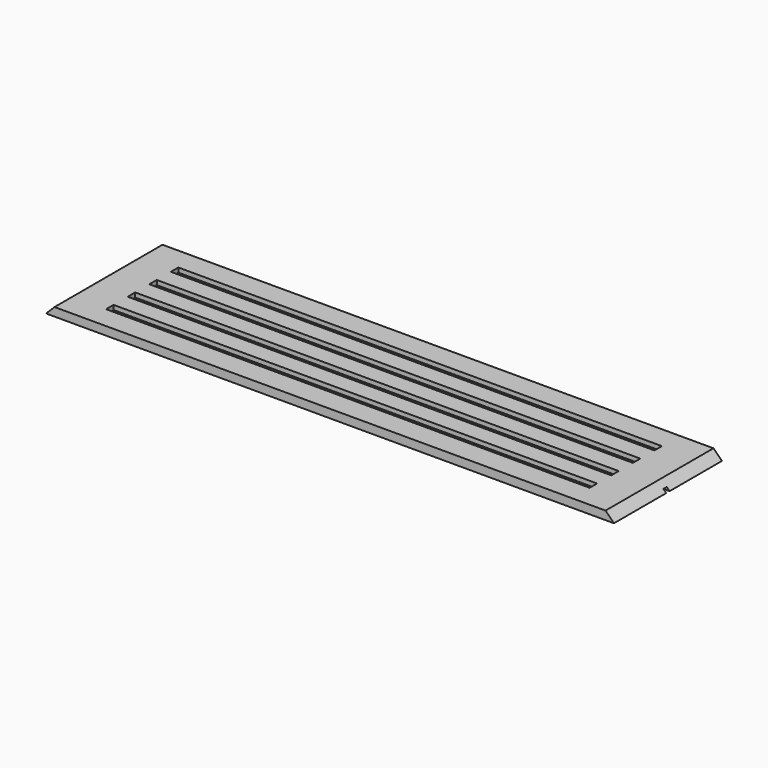
from build123d import *

# Parameters (mm, degrees)
F0_W     = 1282.7
F0_H     = 304.8
F1_DEPTH = 19.05
F2_SIZE  = 19.04999
F3_W     = 1092.2
F3_H     = 21.082
F4_DEPTH = 10.16
F6_DEPTH = 6.35


# Not quite as in the source:
# - a fillet or chamfer is up to 0.001 mm smaller than in the source, because OpenCascade refuses the exact size


with BuildPart() as f1:
    # F0 (on Top) → F1 (new body)
    with BuildSketch(Plane.XY):
        with Locations((362.7905342946, -3.9232242852)):
            Rectangle(F0_W, F0_H)
    extrude(amount=F1_DEPTH)

    # F2 (size 19.05 in the source; OpenCascade refuses exactly that, so slightly less here)
    f2_edges = [f1.edges().sort_by_distance(p)[0] for p in [
        (1004.140534, -3.923224, 19.05),
        (-278.559466, -3.923224, 19.05),
    ]]
    chamfer(f2_edges, length=F2_SIZE)

    # F3 (on face) → F4 (cut)
    with BuildSketch(Plane.XY.offset(19.05)):
        with Locations((362.7905342946, 87.5167757148)):
            Rectangle(F3_W, F3_H)
        with Locations((362.7905342946, 26.5567757148)):
            Rectangle(F3_W, F3_H)
        with Locations((362.7905342946, -34.4032242852)):
            Rectangle(F3_W, F3_H)
        with Locations((362.7905342946, -95.3632242852)):
            Rectangle(F3_W, F3_H)
    extrude(amount=-F4_DEPTH, mode=Mode.SUBTRACT)

    # F5 (on face) → F6 (cut)
    with BuildSketch(Plane(origin=(0, 0, 0), x_dir=(1, 0, 0), z_dir=(0, 0, -1))):
        Polygon((899.3655342946, 105.9042242852), (899.3655342946, -98.0577757148), (908.8905342946, -98.0577757148), (908.8905342946, -0.8392757148), (1004.1405342946, -0.8392757148), (1004.1405342946, 8.6857242852), (908.8905342946, 8.6857242852), (908.8905342946, 105.9042242852), align=None)
        Polygon((-278.5594657054, 8.6857242852), (-278.5594657054, -0.8392757148), (-183.3094657054, -0.8392757148), (-183.3094657054, -98.0577757148), (-173.7844657054, -98.0577757148), (-173.7844657054, 105.9042242852), (-183.3094657054, 105.9042242852), (-183.3094657054, 8.6857242852), align=None)
    extrude(amount=-F6_DEPTH, mode=Mode.SUBTRACT)


solid = f1.part
